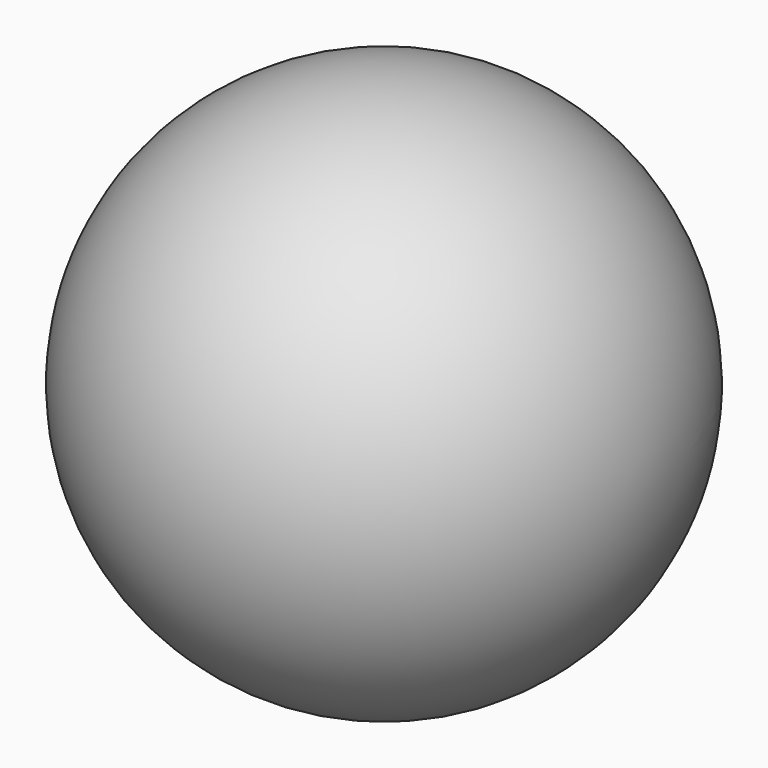
from build123d import *


with BuildPart() as f1:
    # F0 (on Top) → F1 (revolve)
    with BuildSketch(Plane.XY):
        with BuildLine():
            Line((-8.193416521, 0), (51.1346891202, 0))
            ThreePointArc((51.1346891202, 0), (-8.193416521, 59.3281056411), (-67.5215221621, 0))
            Line((-67.5215221621, 0), (-8.193416521, 0))
        make_face()
    revolve(axis=Axis((-8.193416521, 0, 0), (-1, 0, 0)))


solid = f1.part
